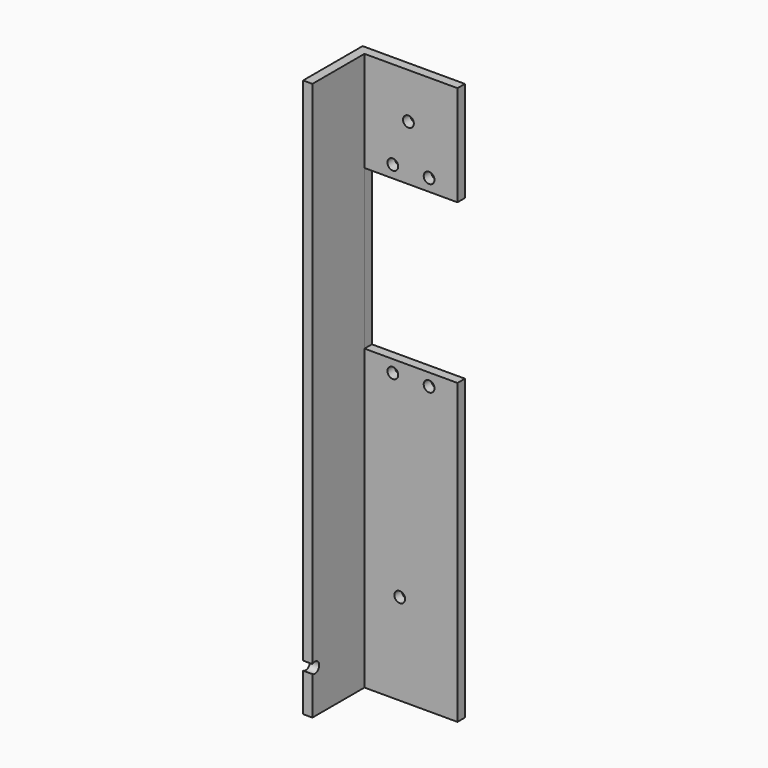
from build123d import *
from build123d import SkipClean  # not in build123d's __all__

# Parameters (mm, degrees)
F0_W     = 2.5400003581
F0_H     = 17.78
F0_H_2   = 2.54
F0_W_2   = 25.3999996419
F1_DEPTH = 152.4
F4_D     = 2.9464
F2_W     = 12.7
F2_H     = 21.717
F5_DEPTH = 2.54
F6_D     = 2.9464
F7_D     = 2.9464
F8_D     = 2.9464
F9_D     = 2.9464
F10_D    = 2.9464
F11_D    = 2.9464


# Not quite as in the source:
# - after a boolean that leaves OpenCascade's solid faulty, fix() repairs it
# - a feature names something its author has since deleted; it is built from what else it names


with BuildPart() as f1:
    # F0 (on Top) → F1 (new body)
    with BuildSketch(Plane.XY):
        with Locations((-9.334868336, -17.2625129279)):
            Rectangle(F0_W, F0_H)
        with Locations((-9.334868336, -7.1025129279)):
            Rectangle(F0_W, F0_H_2)
        with Locations((4.635131664, -7.1025129279)):
            Rectangle(F0_W_2, F0_H_2)
    extrude(amount=F1_DEPTH)

    # F4 (through all)
    with Locations(Plane(origin=(0, -5.8325129279, 0), x_dir=(-1, 0, 0), z_dir=(0, 1, 0))):
        with Locations((0.317868515, 78.1684368849)):
            Hole(F4_D / 2)

    # F2 (on face) → F5 (cut, symmetric)
    with BuildSketch(Plane(origin=(0, -5.8325129279, 0), x_dir=(-1, 0, 0), z_dir=(0, 1, 0))):
        with Locations((1.714868515, 114.0894710903)):
            Rectangle(F2_W, F2_H)
        with Locations((1.714868515, 92.3724710903)):
            Rectangle(F2_W, F2_H)
        with Locations((-10.985131485, 114.0894710903)):
            Rectangle(F2_W, F2_H)
        with Locations((-10.985131485, 92.3724710903)):
            Rectangle(F2_W, F2_H)
    with SkipClean():  # cleaning this boolean's faces spoils the solid; the shape is the same uncleaned
        extrude(amount=F5_DEPTH, both=True, mode=Mode.SUBTRACT)

    # F6 (through all)
    with Locations(Plane(origin=(0, -5.8325129279, 0), x_dir=(-1, 0, 0), z_dir=(0, 1, 0))):
        with Locations((0.317868515, 128.2935052958)):
            Hole(F6_D / 2)

    add(f1.part.fix(), mode=Mode.REPLACE)

    # F7 (through all)
    with Locations(Plane(origin=(0, -5.8325129279, 0), x_dir=(-1, 0, 0), z_dir=(0, 1, 0))):
        with Locations((-9.588131485, 128.2935052958)):
            Hole(F7_D / 2)

    # F8 (through all)
    with Locations(Plane(origin=(0, -5.8325129279, 0), x_dir=(-1, 0, 0), z_dir=(0, 1, 0))):
        with Locations((-9.588131485, 78.1684368849)):
            Hole(F8_D / 2)

    # F9 (through all)
    with Locations(Plane(origin=(0, -5.8325129279, 0), x_dir=(-1, 0, 0), z_dir=(0, 1, 0))):
        with Locations((-3.9381445386, 140.0028020144)):
            Hole(F9_D / 2)

    # F10 (through all)
    with Locations(Plane(origin=(0, -5.8325129279, 0), x_dir=(-1, 0, 0), z_dir=(0, 1, 0))):
        with Locations((-1.56237185, 24.8921643943)):
            Hole(F10_D / 2)

    # F11 (through all)
    with Locations(Plane(origin=(-10.604868515, 0, 0), x_dir=(0, -1, 0), z_dir=(-1, 0, 0))):
        with Locations((25.3072194755, 11.6721792147)):
            Hole(F11_D / 2)


solid = f1.part
